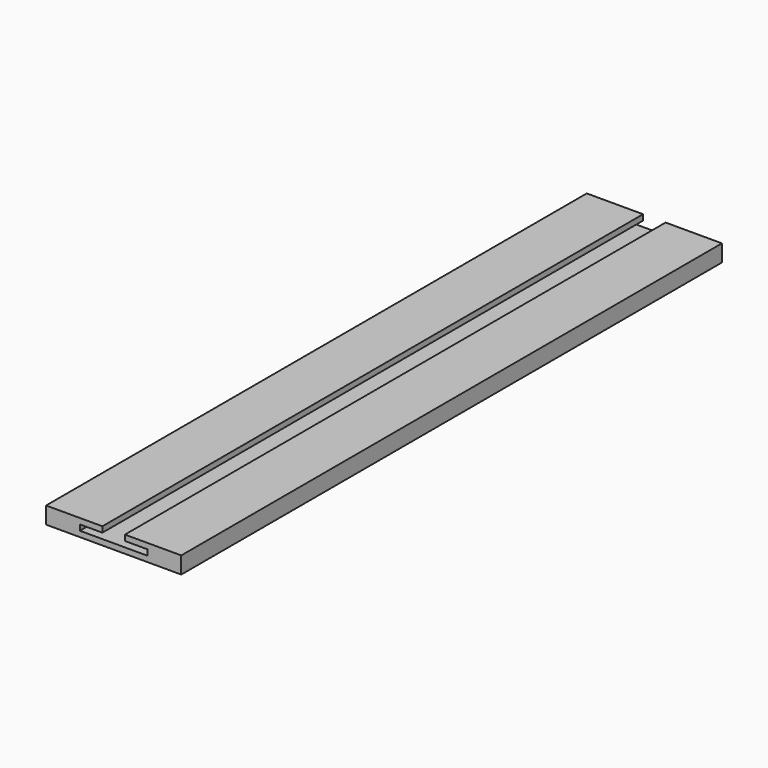
from build123d import *

# Parameters (mm, degrees)
F0_W     = 457.2
F0_H     = 76.2
F0_W_2   = 304.8
F1_DEPTH = 9144


with BuildPart() as f1:
    # F0 (on Front) → F1 (new body)
    with BuildSketch(Plane.XZ):
        with Locations((228.6, 38.1)):
            Rectangle(F0_W, F0_H)
        Polygon((457.2, 0), (0, 0), (0, -76.2), (1828.8, -76.2), (1828.8, 0), (1371.6, 0), align=None)
        with Locations((228.6, 114.3)):
            Rectangle(F0_W, F0_H)
        with Locations((1600.2, 38.1)):
            Rectangle(F0_W, F0_H)
        with Locations((609.6, 114.3)):
            Rectangle(F0_W_2, F0_H)
        with Locations((1600.2, 114.3)):
            Rectangle(F0_W, F0_H)
        with Locations((1219.2, 114.3)):
            Rectangle(F0_W_2, F0_H)
    extrude(amount=F1_DEPTH)


solid = f1.part
